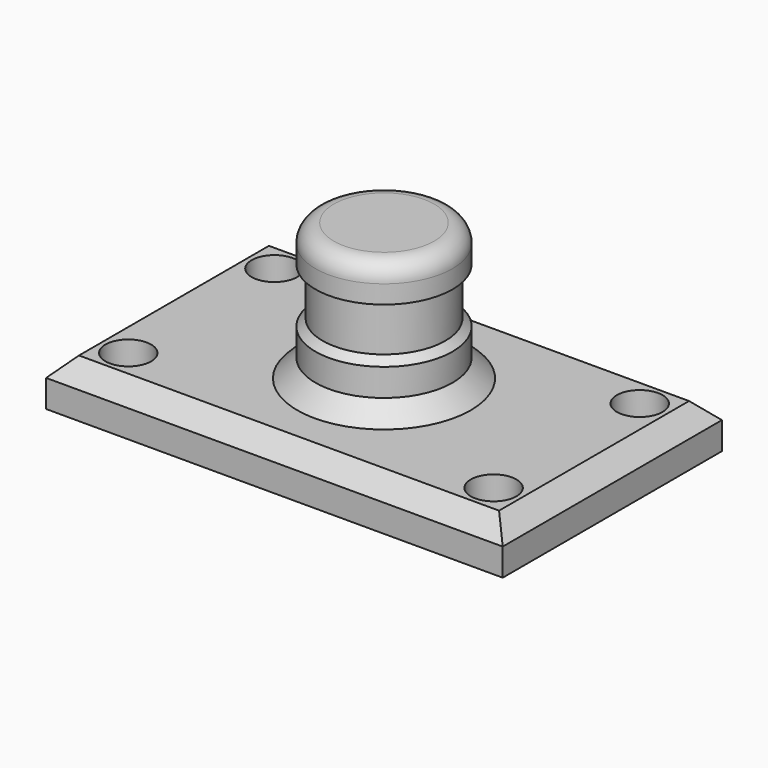
from build123d import *

# Parameters (mm, degrees)
F0_W        = 127
F0_H        = 76.2
F1_DEPTH    = 12.7
F2_R        = 6.35
F3_DEPTH    = 12.701
F4_W        = 19.05
F4_H        = 38.1
F6_W        = 6.35
F6_H        = 10.16
F8_R        = 5.08
F9_S7_R     = 17.0504603439
F9_T8_DEPTH = 29
F10_SIZE    = 5.08


# Not quite as in the source:
# - a fillet or chamfer that OpenCascade refuses, or shapes differently, is made with other operations: its cross-section is extruded or revolved along the edge and cut away or added


with BuildPart() as f1:
    # F0 (on Top) → F1 (new body)
    with BuildSketch(Plane.XY):
        Rectangle(F0_W, F0_H)
    extrude(amount=F1_DEPTH)

    # F2 (on face) → F3 (cut, through all)
    with BuildSketch(Plane.XY.offset(12.7)):
        with Locations((50.8, -25.4)):
            Circle(F2_R)
        with Locations((50.8, 25.4)):
            Circle(F2_R)
        with Locations((-50.8, 25.4)):
            Circle(F2_R)
        with Locations((-50.8, -25.4)):
            Circle(F2_R)
    extrude(amount=-F3_DEPTH, mode=Mode.SUBTRACT)

    # F4 (on Front) → F5 (revolve)
    with BuildSketch(Plane.XZ):
        with Locations((9.525, 31.75)):
            Rectangle(F4_W, F4_H)
    revolve(axis=Axis((0, 0, 31.75), (0, 0, 1)))

    # F6 (on Front) → F7 (revolve, cut)
    with BuildSketch(Plane.XZ):
        with Locations((20.2254603439, 35.56)):
            Rectangle(F6_W, F6_H)
    revolve(axis=Axis((0, 0, 50.8), (0, 0, 1)), mode=Mode.SUBTRACT)

    # F8
    f8_edges = [f1.edges().sort_by_distance(p)[0] for p in [
        (-19.05, 0, 50.8),
    ]]
    fillet(f8_edges, radius=F8_R)

    # F9: chamfer of 5.08 on 3 edges, made by hand

    # F9_s1 → F9_t2 (revolve)
    with BuildSketch(Plane.XZ):
        Polygon((19.05, 17.78), (24.13, 12.7), (19.05, 12.7), align=None)
    revolve(axis=Axis((0, 0, 12.7), (0, 0, 1)))


with BuildPart() as f9_tool4:
    # F9_s5 → F9_t6 (revolve)
    with BuildSketch(Plane.XZ):
        Polygon((13.97, 30.48), (19.05, 25.4), (19.05, 30.48), align=None)
    revolve(axis=Axis((0, 0, 30.48), (0, 0, 1)))

    # F9_s7 → F9_t8 (cut, symmetric)
    with BuildSketch(Plane.XY.offset(27.9)):
        Circle(F9_S7_R)
    extrude(amount=F9_T8_DEPTH, both=True, mode=Mode.SUBTRACT)


with BuildPart() as f1_1:
    add(f1.part)

    # F9_t3: cut F9_tool4
    add(f9_tool4.part, mode=Mode.SUBTRACT)

    # F10
    f10_edges = [f1_1.edges().sort_by_distance(p)[0] for p in [
        (0, -38.1, 12.7),
        (63.5, 0, 12.7),
        (0, 38.1, 12.7),
        (-63.5, 0, 12.7),
    ]]
    chamfer(f10_edges, length=F10_SIZE)


solid = f1_1.part
